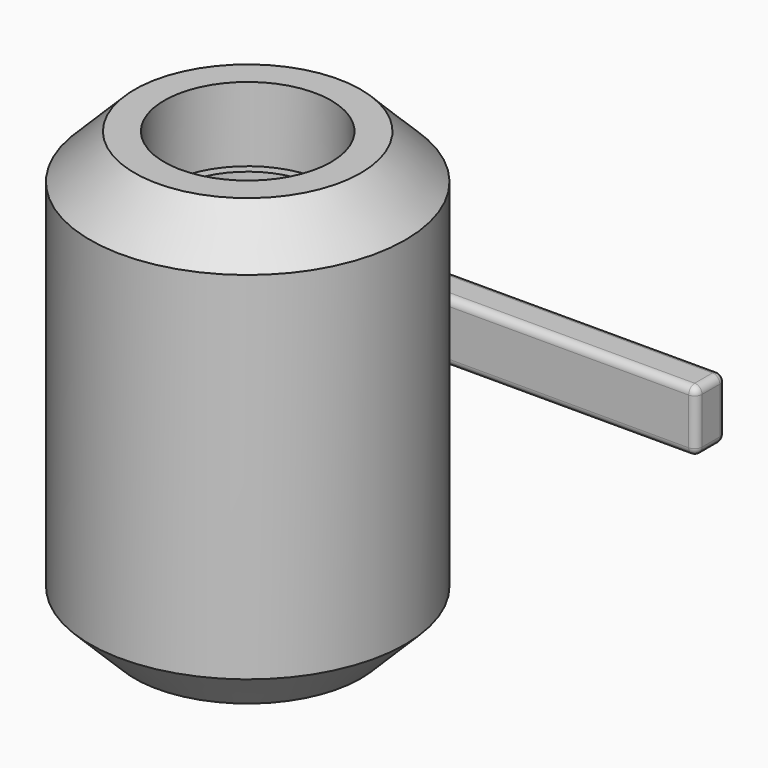
from build123d import *

# Parameters (mm, degrees)
F0_R          = 14.2875
F0_R_2        = 12.7
F2_DEPTH      = 50.8
F3_R          = 26.9875
F3_R_2        = 14.2875
F4_DEPTH      = 63.5
F4_DEPTH_BACK = 12.7
F5_SIZE       = 7.62
F7_START      = -26.67
F6_W          = 64.1522035003
F6_H          = 10.4847997427
F7_DEPTH      = 6.35
F8_R          = 1.26999


# Not quite as in the source:
# - a fillet or chamfer is up to 0.001 mm smaller than in the source, because OpenCascade refuses the exact size
# - a feature names something its author has since deleted; it is built from what else it names


with BuildPart() as f2:
    # F0 (on Top) → F2 (new body)
    with BuildSketch(Plane.XY):
        Circle(F0_R)
        Circle(F0_R_2, mode=Mode.SUBTRACT)
    extrude(amount=F2_DEPTH)

    # F3 (on face) → F4 (join, two sides)
    with BuildSketch(Plane.XY) as f4_sk:
        Circle(F3_R)
        Circle(F3_R_2, mode=Mode.SUBTRACT)
    extrude(amount=F4_DEPTH)
    extrude(f4_sk.sketch, amount=-F4_DEPTH_BACK)

    # F5
    f5_edges = [f2.edges().sort_by_distance(p)[0] for p in [
        (-26.9875, 0, 63.5),
        (-26.9875, 0, -12.7),
    ]]
    chamfer(f5_edges, length=F5_SIZE)

    # F6 (on Front) → F7 (join)
    with BuildSketch(Plane.XZ.offset(F7_START)):
        with Locations((23.3749561012, 26.5372619033)):
            Rectangle(F6_W, F6_H)
    extrude(amount=-F7_DEPTH)

    # F8 (radius 1.27 in the source; OpenCascade refuses exactly that, so slightly less here)
    f8_edges = [f2.edges().sort_by_distance(p)[0] for p in [
        (23.374956, 33.02, 31.779662),
        (23.374956, 33.02, 21.294862),
        (-8.701146, 33.02, 26.537262),
        (29.789279, 26.67, 21.294862),
        (29.789279, 26.67, 31.779662),
        (55.451058, 26.67, 26.537262),
        (55.451058, 29.845, 31.779662),
        (55.451058, 33.02, 26.537262),
        (55.451058, 29.845, 21.294862),
    ]]
    fillet(f8_edges, radius=F8_R)


solid = f2.part
